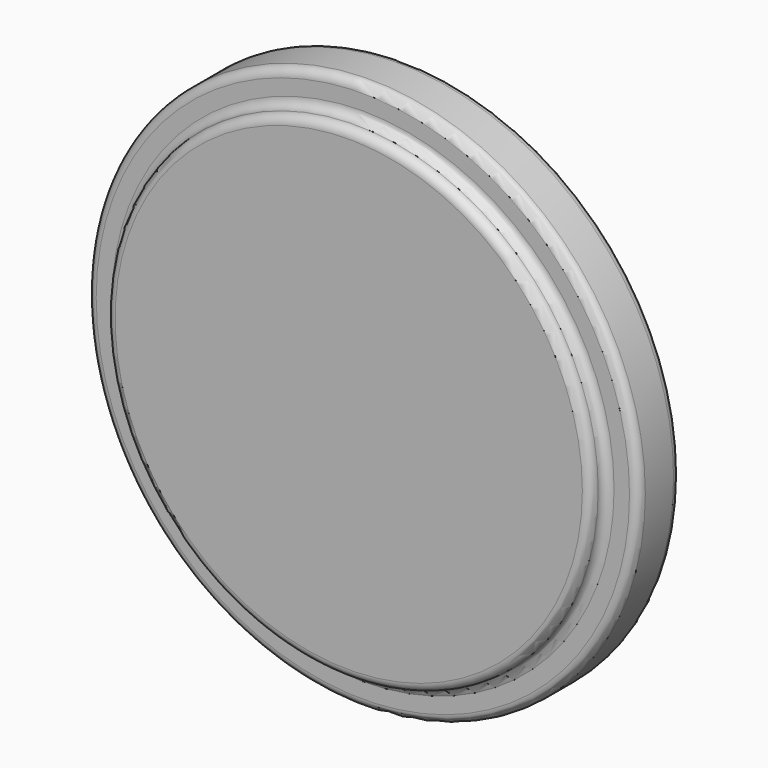
from build123d import *

# Parameters (mm, degrees)
F0_R     = 5.5
F1_DEPTH = 1.6
F0_R_2   = 6.25
F2_DEPTH = 1.2
F3_R     = 0.19999


# Not quite as in the source:
# - a fillet or chamfer is up to 0.001 mm smaller than in the source, because OpenCascade refuses the exact size


with BuildPart() as f1:
    # F0 (on Front) → F1 (new body)
    with BuildSketch(Plane.XZ):
        with Locations((6.25, 6.25)):
            Circle(F0_R)
    extrude(amount=F1_DEPTH)

    # F0 (on Front) → F2 (join)
    with BuildSketch(Plane.XZ):
        with Locations((6.25, 6.25)):
            Circle(F0_R_2)
        with Locations((6.25, 6.25)):
            Circle(F0_R, mode=Mode.SUBTRACT)
    extrude(amount=F2_DEPTH)

    # F3 (radius 0.2 in the source; OpenCascade refuses exactly that, so slightly less here)
    f3_edges = [f1.edges().sort_by_distance(p)[0] for p in [
        (0.75, -1.6, 6.25),
        (12.5, -0.6, 6.25),
        (0, 0, 6.25),
        (0, -1.2, 6.25),
        (0.75, -1.2, 6.25),
        (11.75, -1.4, 6.25),
    ]]
    fillet(f3_edges, radius=F3_R)


solid = f1.part
